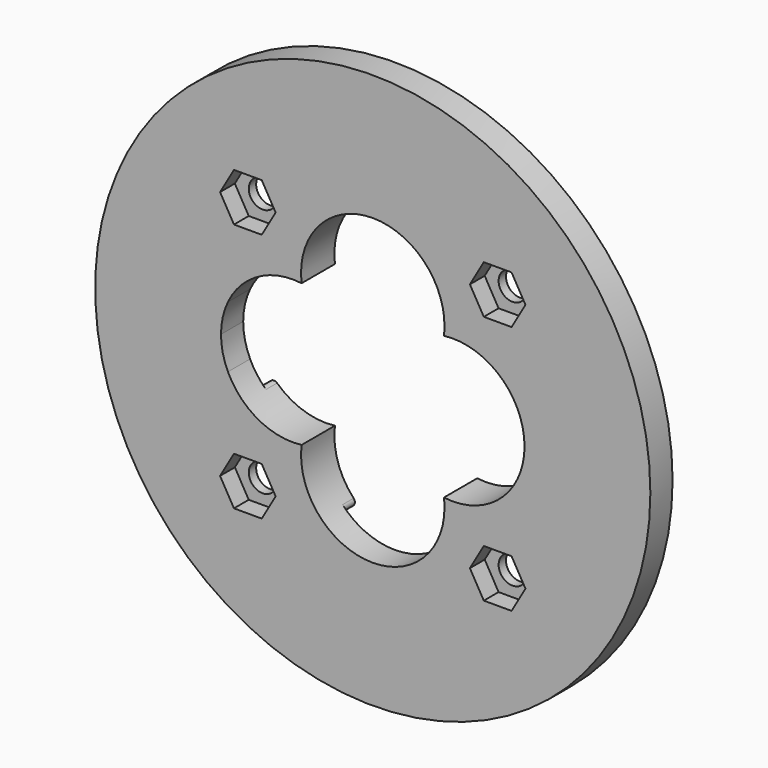
from build123d import *

# Parameters (mm, degrees)
F0_R        = 30
F1_DEPTH    = 3
F4_DEPTH    = 1.5
F5_T1_DEPTH = 9.1064563612
F2_R        = 1.5
F3_DEPTH    = 2
F6_DEPTH    = 25


# Not quite as in the source:
# - a fillet or chamfer that OpenCascade refuses, or shapes differently, is made with other operations: its cross-section is extruded or revolved along the edge and cut away or added


with BuildPart() as f1:
    # F0 (on Front) → F1 (new body)
    with BuildSketch(Plane.XZ):
        Circle(F0_R)
        with BuildLine():
            ThreePointArc((0, 16.4), (11.5965512115, 11.5965512115), (16.4, 0))
            ThreePointArc((16.4, 0), (11.5965511405, -11.5965512824), (-2.007e-07, -16.4))
            ThreePointArc((-2.007e-07, -16.4), (-11.5965512889, -11.596551134), (-16.4, 1.83e-08))
            ThreePointArc((-16.4, 1.83e-08), (-11.596551205, 11.5965512179), (0, 16.4))
        make_face(mode=Mode.SUBTRACT)
        with BuildLine():
            ThreePointArc((7.6903565933, 7.6903565933), (12.3769167702, 6.7950416767), (15.650867052, 3.3242082546))
            ThreePointArc((15.650867052, 3.3242082546), (11.313708499, 11.313708499), (3.3242082546, 15.650867052))
            ThreePointArc((3.3242082546, 15.650867052), (6.5507676639, 12.7912489678), (7.75, 8.65))
            ThreePointArc((7.75, 8.65), (7.7350747766, 8.1692524561), (7.6903565933, 7.6903565933))
        make_face()
        with BuildLine():
            ThreePointArc((3.3242082546, -15.650867052), (11.313708499, -11.313708499), (15.650867052, -3.3242082546))
            ThreePointArc((15.650867052, -3.3242082546), (12.3769167702, -6.7950416767), (7.6903565933, -7.6903565933))
            ThreePointArc((7.6903565933, -7.6903565933), (7.7350747766, -8.1692524561), (7.75, -8.65))
            ThreePointArc((7.75, -8.65), (6.5507676639, -12.7912489678), (3.3242082546, -15.650867052))
        make_face()
        with BuildLine():
            ThreePointArc((-7.6903565933, 7.6903565933), (-6.7950416767, 12.3769167702), (-3.3242082546, 15.650867052))
            ThreePointArc((-3.3242082546, 15.650867052), (-11.313708499, 11.313708499), (-15.650867052, 3.3242082546))
            ThreePointArc((-15.650867052, 3.3242082546), (-12.3769167702, 6.7950416767), (-7.6903565933, 7.6903565933))
        make_face()
        with BuildLine():
            ThreePointArc((-15.650867052, -3.3242082546), (-11.313708499, -11.313708499), (-3.3242082546, -15.650867052))
            ThreePointArc((-3.3242082546, -15.650867052), (-6.7950416767, -12.3769167702), (-7.6903565933, -7.6903565933))
            ThreePointArc((-7.6903565933, -7.6903565933), (-12.3769167702, -6.7950416767), (-15.650867052, -3.3242082546))
        make_face()
        with BuildLine():
            ThreePointArc((15.650867052, 3.3242082546), (16.2103974649, 1.7037870094), (16.4, 0))
            ThreePointArc((16.4, 0), (11.5965512115, 11.5965512115), (0, 16.4))
            ThreePointArc((0, 16.4), (1.7037870094, 16.2103974649), (3.3242082546, 15.650867052))
            ThreePointArc((3.3242082546, 15.650867052), (11.313708499, 11.313708499), (15.650867052, 3.3242082546))
        make_face()
        with BuildLine():
            ThreePointArc((-2.007e-07, -16.4), (11.5965511405, -11.5965512824), (16.4, 0))
            ThreePointArc((16.4, 0), (16.2103974649, -1.7037870094), (15.650867052, -3.3242082546))
            ThreePointArc((15.650867052, -3.3242082546), (11.313708499, -11.313708499), (3.3242082546, -15.650867052))
            ThreePointArc((3.3242082546, -15.650867052), (1.7037869115, -16.2103974869), (-2.007e-07, -16.4))
        make_face()
        with BuildLine():
            ThreePointArc((-3.3242082546, 15.650867052), (-1.7037870094, 16.2103974649), (0, 16.4))
            ThreePointArc((0, 16.4), (-11.596551205, 11.5965512179), (-16.4, 1.83e-08))
            ThreePointArc((-16.4, 1.83e-08), (-16.2103974628, 1.7037870183), (-15.650867052, 3.3242082546))
            ThreePointArc((-15.650867052, 3.3242082546), (-11.313708499, 11.313708499), (-3.3242082546, 15.650867052))
        make_face()
        with BuildLine():
            ThreePointArc((-16.4, 1.83e-08), (-11.5965512889, -11.596551134), (-2.007e-07, -16.4))
            ThreePointArc((-2.007e-07, -16.4), (-1.7037871073, -16.2103974428), (-3.3242082546, -15.650867052))
            ThreePointArc((-3.3242082546, -15.650867052), (-11.313708499, -11.313708499), (-15.650867052, -3.3242082546))
            ThreePointArc((-15.650867052, -3.3242082546), (-16.2103974669, -1.7037870005), (-16.4, 1.83e-08))
        make_face()
    extrude(amount=F1_DEPTH)

    # F0 (on Front) → F4 (join)
    with BuildSketch(Plane.XZ):
        with BuildLine():
            ThreePointArc((7.6903565933, 7.6903565933), (12.3769167702, 6.7950416767), (15.650867052, 3.3242082546))
            ThreePointArc((15.650867052, 3.3242082546), (11.313708499, 11.313708499), (3.3242082546, 15.650867052))
            ThreePointArc((3.3242082546, 15.650867052), (6.5507676639, 12.7912489678), (7.75, 8.65))
            ThreePointArc((7.75, 8.65), (7.7350747766, 8.1692524561), (7.6903565933, 7.6903565933))
        make_face()
        with BuildLine():
            ThreePointArc((3.3242082546, -15.650867052), (11.313708499, -11.313708499), (15.650867052, -3.3242082546))
            ThreePointArc((15.650867052, -3.3242082546), (12.3769167702, -6.7950416767), (7.6903565933, -7.6903565933))
            ThreePointArc((7.6903565933, -7.6903565933), (7.7350747766, -8.1692524561), (7.75, -8.65))
            ThreePointArc((7.75, -8.65), (6.5507676639, -12.7912489678), (3.3242082546, -15.650867052))
        make_face()
        with BuildLine():
            ThreePointArc((-7.6903565933, 7.6903565933), (-6.7950416767, 12.3769167702), (-3.3242082546, 15.650867052))
            ThreePointArc((-3.3242082546, 15.650867052), (-11.313708499, 11.313708499), (-15.650867052, 3.3242082546))
            ThreePointArc((-15.650867052, 3.3242082546), (-12.3769167702, 6.7950416767), (-7.6903565933, 7.6903565933))
        make_face()
        with BuildLine():
            ThreePointArc((-15.650867052, -3.3242082546), (-11.313708499, -11.313708499), (-3.3242082546, -15.650867052))
            ThreePointArc((-3.3242082546, -15.650867052), (-6.7950416767, -12.3769167702), (-7.6903565933, -7.6903565933))
            ThreePointArc((-7.6903565933, -7.6903565933), (-12.3769167702, -6.7950416767), (-15.650867052, -3.3242082546))
        make_face()
    extrude(amount=-F4_DEPTH)

    # F5: fillet of radius 0.5 on 8 edges, made by hand

    # F5_s2 → F5_t1 (cut)
    with BuildSketch(Plane.XZ.offset(-9.1064563612)):
        with BuildLine():
            ThreePointArc((-6.2268118052, -14.738616446), (-5.6223691009, -14.5644243012), (-5.6666346068, -13.936941671))
            ThreePointArc((-5.6666346068, -13.936941671), (-4.5763739896, -14.9045424379), (-3.3242082546, -15.650867052))
            ThreePointArc((-3.3242082546, -15.650867052), (-4.7972436187, -15.263893791), (-6.2268118052, -14.738616446))
        make_face()
        with BuildLine():
            ThreePointArc((6.2268118052, -14.738616446), (5.6223691009, -14.5644243012), (5.6666346068, -13.936941671))
            ThreePointArc((5.6666346068, -13.936941671), (4.5763739896, -14.9045424379), (3.3242082546, -15.650867052))
            ThreePointArc((3.3242082546, -15.650867052), (4.7972436187, -15.263893791), (6.2268118052, -14.738616446))
        make_face()
        with BuildLine():
            ThreePointArc((13.936941671, 5.6666346068), (14.5644243012, 5.6223691009), (14.738616446, 6.2268118052))
            ThreePointArc((14.738616446, 6.2268118052), (15.263893791, 4.7972436187), (15.650867052, 3.3242082546))
            ThreePointArc((15.650867052, 3.3242082546), (14.9045424379, 4.5763739896), (13.936941671, 5.6666346068))
        make_face()
        with BuildLine():
            ThreePointArc((13.936941671, -5.6666346068), (14.5644243012, -5.6223691009), (14.738616446, -6.2268118052))
            ThreePointArc((14.738616446, -6.2268118052), (15.263893791, -4.7972436187), (15.650867052, -3.3242082546))
            ThreePointArc((15.650867052, -3.3242082546), (14.9045424379, -4.5763739896), (13.936941671, -5.6666346068))
        make_face()
        with BuildLine():
            ThreePointArc((-13.936941671, 5.6666346068), (-14.5644243012, 5.6223691009), (-14.738616446, 6.2268118052))
            ThreePointArc((-14.738616446, 6.2268118052), (-15.263893791, 4.7972436187), (-15.650867052, 3.3242082546))
            ThreePointArc((-15.650867052, 3.3242082546), (-14.9045424379, 4.5763739896), (-13.936941671, 5.6666346068))
        make_face()
        with BuildLine():
            ThreePointArc((-14.738616446, -6.2268118052), (-14.5644243012, -5.6223691009), (-13.936941671, -5.6666346068))
            ThreePointArc((-13.936941671, -5.6666346068), (-14.9045424379, -4.5763739896), (-15.650867052, -3.3242082546))
            ThreePointArc((-15.650867052, -3.3242082546), (-15.263893791, -4.7972436187), (-14.738616446, -6.2268118052))
        make_face()
        with BuildLine():
            ThreePointArc((6.2268118052, 14.738616446), (5.6223691009, 14.5644243012), (5.6666346068, 13.936941671))
            ThreePointArc((5.6666346068, 13.936941671), (4.5763739896, 14.9045424379), (3.3242082546, 15.650867052))
            ThreePointArc((3.3242082546, 15.650867052), (4.7972436187, 15.263893791), (6.2268118052, 14.738616446))
        make_face()
        with BuildLine():
            ThreePointArc((-6.2268118052, 14.738616446), (-5.6223691009, 14.5644243012), (-5.6666346068, 13.936941671))
            ThreePointArc((-5.6666346068, 13.936941671), (-4.5763739896, 14.9045424379), (-3.3242082546, 15.650867052))
            ThreePointArc((-3.3242082546, 15.650867052), (-4.7972436187, 15.263893791), (-6.2268118052, 14.738616446))
        make_face()
    extrude(amount=F5_T1_DEPTH, mode=Mode.SUBTRACT)

    # F2 (on face) → F3 (cut)
    with BuildSketch(Plane.XZ.offset(3)):
        Polygon((-15.0011106999, 10.9), (-11.9988893001, 10.9), (-10.4977786002, 13.5), (-11.9988893001, 16.1), (-15.0011106999, 16.1), (-16.5022213998, 13.5), align=None)
        with Locations((-13.5, 13.5)):
            Circle(F2_R, mode=Mode.SUBTRACT)
        Polygon((11.9988893001, 10.9), (15.0011106999, 10.9), (16.5022213998, 13.5), (15.0011106999, 16.1), (11.9988893001, 16.1), (10.4977786002, 13.5), align=None)
        with Locations((13.5, 13.5)):
            Circle(F2_R, mode=Mode.SUBTRACT)
        Polygon((-11.9988893001, -10.9), (-15.0011106999, -10.9), (-16.5022213998, -13.5), (-15.0011106999, -16.1), (-11.9988893001, -16.1), (-10.4977786002, -13.5), align=None)
        with Locations((-13.5, -13.5)):
            Circle(F2_R, mode=Mode.SUBTRACT)
        Polygon((15.0011106999, -10.9), (11.9988893001, -10.9), (10.4977786002, -13.5), (11.9988893001, -16.1), (15.0011106999, -16.1), (16.5022213998, -13.5), align=None)
        with Locations((13.5, -13.5)):
            Circle(F2_R, mode=Mode.SUBTRACT)
    extrude(amount=-F3_DEPTH, mode=Mode.SUBTRACT)

    # F2 (on face) → F6 (cut)
    with BuildSketch(Plane.XZ.offset(3)):
        with Locations((-13.5, 13.5)):
            Circle(F2_R)
        with Locations((13.5, 13.5)):
            Circle(F2_R)
        with Locations((13.5, -13.5)):
            Circle(F2_R)
        with Locations((-13.5, -13.5)):
            Circle(F2_R)
    extrude(amount=-F6_DEPTH, mode=Mode.SUBTRACT)


solid = f1.part
